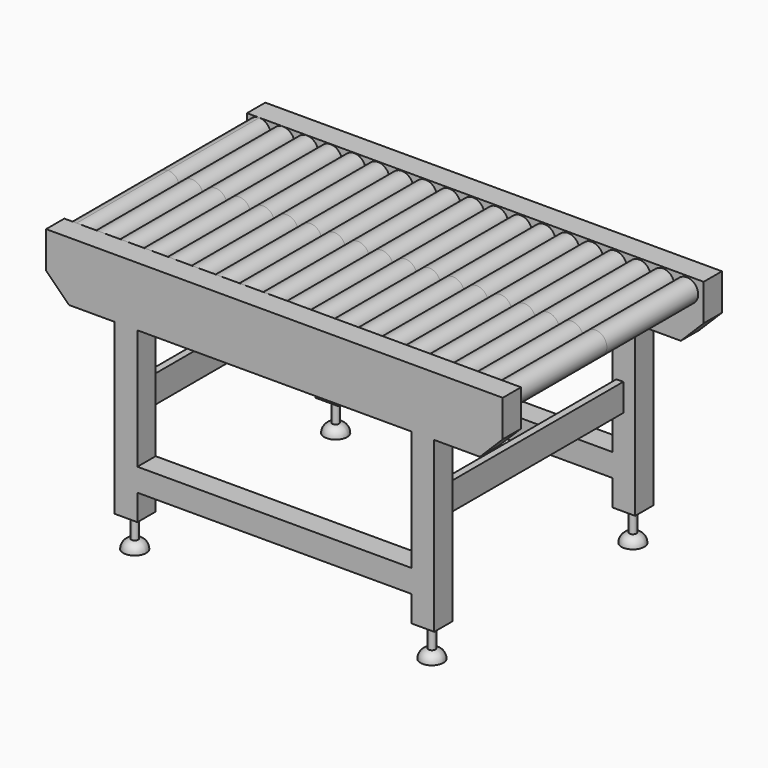
from build123d import *

# Parameters (mm, degrees)
F0_W      = 600
F0_H      = 263.0605769157
F1_DEPTH  = 50
F2_SIZE   = 50
F3_SIZE   = 50
F4_R      = 25
F5_DEPTH  = 250
F6_R      = 7.5
F7_DEPTH  = 50
F8_W      = 15
F8_H      = 60
F9_DEPTH  = 250
F10_R     = 25
F10_R_2   = 7.5
F11_DEPTH = 20


# Not quite as in the source:
# - a fillet or chamfer that OpenCascade refuses, or shapes differently, is made with other operations: its cross-section is extruded or revolved along the edge and cut away or added


with BuildPart() as f1:
    # F0 (on Front) → F1 (new body)
    with BuildSketch(Plane.XZ):
        Polygon((505.5267233402, 46.2662550807), (-494.4732766598, 46.2662550807), (-494.4732766598, -83.7337449193), (-344.4732766598, -83.7337449193), (-344.4732766598, -453.7337449193), (-294.4732766598, -453.7337449193), (-294.4732766598, -396.794321835), (305.5267233402, -396.794321835), (305.5267233402, -453.7337449193), (355.5267233402, -453.7337449193), (355.5267233402, -83.7337449193), (505.5267233402, -83.7337449193), align=None)
        with Locations((5.5267233402, -215.2640333772)):
            Rectangle(F0_W, F0_H, mode=Mode.SUBTRACT)
    extrude(amount=F1_DEPTH)

    # F2
    f2_edges = [f1.edges().sort_by_distance(p)[0] for p in [
        (505.526723, -25, -83.733745),
    ]]
    chamfer(f2_edges, length=F2_SIZE)

    # F3
    f3_edges = [f1.edges().sort_by_distance(p)[0] for p in [
        (-494.473277, -25, -83.733745),
    ]]
    chamfer(f3_edges, length=F3_SIZE)

    # F4 (on face) → F5 (join)
    with BuildSketch(Plane.XZ.offset(50)):
        with BuildLine():
            ThreePointArc((-467.4732766598, 46.2662550807), (-485.1509461895, 3.588585551), (-442.4732766598, 21.2662550807))
            ThreePointArc((-442.4732766598, 21.2662550807), (-449.7956071302, 38.9439246104), (-467.4732766598, 46.2662550807))
        make_face()
        with Locations((-415.4736002376, 21.0828103085)):
            Circle(F4_R)
        with Locations((-363.4739238154, 20.8993655363)):
            Circle(F4_R)
        with Locations((-311.4742473932, 20.7159207642)):
            Circle(F4_R)
        with Locations((-259.474570971, 20.532475992)):
            Circle(F4_R)
        with Locations((-207.4748945487, 20.3490312198)):
            Circle(F4_R)
        with Locations((-155.4752181265, 20.1655864476)):
            Circle(F4_R)
        with Locations((-103.4755417043, 19.9821416755)):
            Circle(F4_R)
        with Locations((-51.4758652821, 19.7986969033)):
            Circle(F4_R)
        with Locations((0.5238111401, 19.6152521311)):
            Circle(F4_R)
        with Locations((52.5234875624, 19.4318073589)):
            Circle(F4_R)
        with Locations((104.5231639846, 19.2483625868)):
            Circle(F4_R)
        with Locations((156.5228404068, 19.0649178146)):
            Circle(F4_R)
        with Locations((208.522516829, 18.8814730424)):
            Circle(F4_R)
        with Locations((260.5221932512, 18.6980282702)):
            Circle(F4_R)
        with Locations((312.5218696735, 18.5145834981)):
            Circle(F4_R)
        with Locations((364.5215460957, 18.3311387259)):
            Circle(F4_R)
        with Locations((416.5212225179, 18.1476939537)):
            Circle(F4_R)
        with Locations((468.5208989401, 17.9642491815)):
            Circle(F4_R)
    extrude(amount=F5_DEPTH)

    # F6 (on face) → F7 (join)
    with BuildSketch(Plane(origin=(0, 0, -453.7337449193), x_dir=(1, 0, 0), z_dir=(0, 0, -1))):
        with Locations((-320.3388154507, 25)):
            Circle(F6_R)
        with Locations((330.5267233402, 25)):
            Circle(F6_R)
    extrude(amount=F7_DEPTH)

    # F8 (on face) → F9 (join)
    with BuildSketch(Plane.XZ.offset(50)):
        with Locations((-321.9732766598, -233.7337449193)):
            Rectangle(F8_W, F8_H)
        with Locations((321.9732766598, -233.7337449193)):
            Rectangle(F8_W, F8_H)
    extrude(amount=F9_DEPTH)

    # F10 (on face) → F11 (join)
    with BuildSketch(Plane(origin=(0, 0, -503.7337449193), x_dir=(1, 0, 0), z_dir=(0, 0, -1))):
        with Locations((-320.3388154507, 25)):
            Circle(F10_R)
        with Locations((-320.3388154507, 25)):
            Circle(F10_R_2, mode=Mode.SUBTRACT)
        with Locations((-320.3388154507, 25)):
            Circle(F10_R_2)
        with Locations((330.5267233402, 25)):
            Circle(F10_R)
    extrude(amount=F11_DEPTH)

    # F12: fillet of radius 20 on 2 edges, made by hand

    # F12_s1 → F12_t2 (revolve, cut)
    with BuildSketch(Plane.XZ.offset(25)):
        with BuildLine():
            ThreePointArc((-295.3388154507, -523.5768797523), (-300.3388154507, -510.348123197), (-312.8388154507, -503.7337449193))
            Line((-312.8388154507, -503.7337449193), (-295.3388154507, -503.7337449193))
            Line((-295.3388154507, -503.7337449193), (-295.3388154507, -523.5768797523))
        make_face()
    revolve(axis=Axis((-320.3388154507, -25, -503.7337449193), (0, 0, -1)), mode=Mode.SUBTRACT)

    # F12_s3 → F12_t4 (revolve, cut)
    with BuildSketch(Plane.XZ.offset(25)):
        with BuildLine():
            ThreePointArc((338.0267233402, -503.7337449193), (350.5267233402, -510.348123197), (355.5267233402, -523.5768797523))
            Line((355.5267233402, -523.5768797523), (355.5267233402, -503.7337449193))
            Line((355.5267233402, -503.7337449193), (338.0267233402, -503.7337449193))
        make_face()
    revolve(axis=Axis((330.5267233402, -25, -503.7337449193), (0, 0, -1)), mode=Mode.SUBTRACT)

    # F13: F1 across face


with BuildPart() as f1_1:
    add(f1.part)
    add(f1.part.mirror(Plane(origin=(104.5231639846, -300, 19.2483625868), x_dir=(1, 0, 0), z_dir=(0, -1, 0))))


solid = f1_1.part
